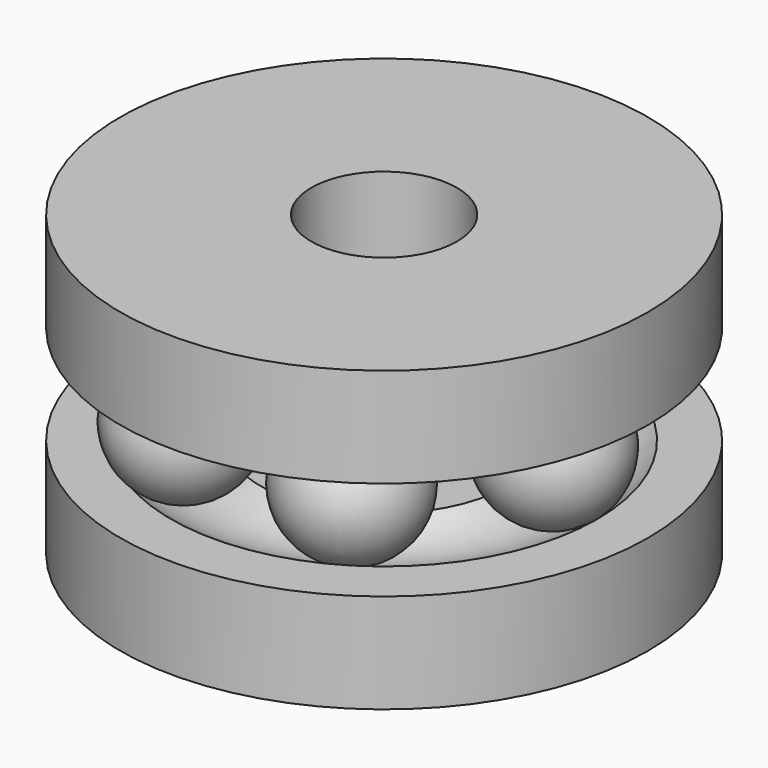
from build123d import *

# Parameters (mm, degrees)
F4_COUNT = 6


with BuildPart() as f1:
    # F0 (on Front) → F1 (revolve)
    with BuildSketch(Plane.XZ):
        with BuildLine():
            Line((0, 12.9999994), (0, 0))
            Line((0, 0), (25.0000008, 0))
            Line((25.0000008, 0), (25.0000008, 12.9999994))
            Line((25.0000008, 12.9999994), (18.3576743155, 12.9999994))
            ThreePointArc((18.3576743155, 12.9999994), (12.5000004, 10.75001152), (6.6423264845, 12.9999994))
            Line((6.6423264845, 12.9999994), (0, 12.9999994))
        make_face()
    revolve(axis=Axis((-9.525, 0, 14.372562758), (0, 0, 1)))


with BuildPart() as f3:
    # F2 (on Front) → F3 (revolve)
    with BuildSketch(Plane.XZ):
        with BuildLine():
            Line((21.25000068, 19.5000118), (3.75000012, 19.5000118))
            ThreePointArc((3.75000012, 19.5000118), (12.5000004, 10.75001152), (21.25000068, 19.5000118))
        make_face()
    revolve(axis=Axis((12.5000004, 0, 19.5000118), (1, 0, 0)))


with BuildPart() as f4_1:
    # F4: instance of F3
    add(f3.part.rotate(Axis((-9.525, 0, 12.9999994), (0, 0, -1)), 1 * 360 / F4_COUNT))


with BuildPart() as f4_2:
    # F4: instance of F3
    add(f3.part.rotate(Axis((-9.525, 0, 12.9999994), (0, 0, -1)), 2 * 360 / F4_COUNT))


with BuildPart() as f4_3:
    # F4: instance of F3
    add(f3.part.rotate(Axis((-9.525, 0, 12.9999994), (0, 0, -1)), 3 * 360 / F4_COUNT))


with BuildPart() as f4_4:
    # F4: instance of F3
    add(f3.part.rotate(Axis((-9.525, 0, 12.9999994), (0, 0, -1)), 4 * 360 / F4_COUNT))


with BuildPart() as f4_5:
    # F4: instance of F3
    add(f3.part.rotate(Axis((-9.525, 0, 12.9999994), (0, 0, -1)), 5 * 360 / F4_COUNT))


with BuildPart() as f6:
    # F5 (on Front) → F6 (revolve)
    with BuildSketch(Plane.XZ):
        with BuildLine():
            Line((0, 39.0000236), (0, 26.0000242))
            Line((0, 26.0000242), (6.6423264845, 26.0000242))
            ThreePointArc((6.6423264845, 26.0000242), (12.5000004, 28.25001208), (18.3576743155, 26.0000242))
            Line((18.3576743155, 26.0000242), (25.0000008, 26.0000242))
            Line((25.0000008, 26.0000242), (25.0000008, 39.0000236))
            Line((25.0000008, 39.0000236), (0, 39.0000236))
        make_face()
    revolve(axis=Axis((-9.525, 0, 20.579790572), (0, 0, 1)))


solid = Compound([f1.part, f3.part, f4_1.part, f4_2.part, f4_3.part, f4_4.part, f4_5.part, f6.part])
